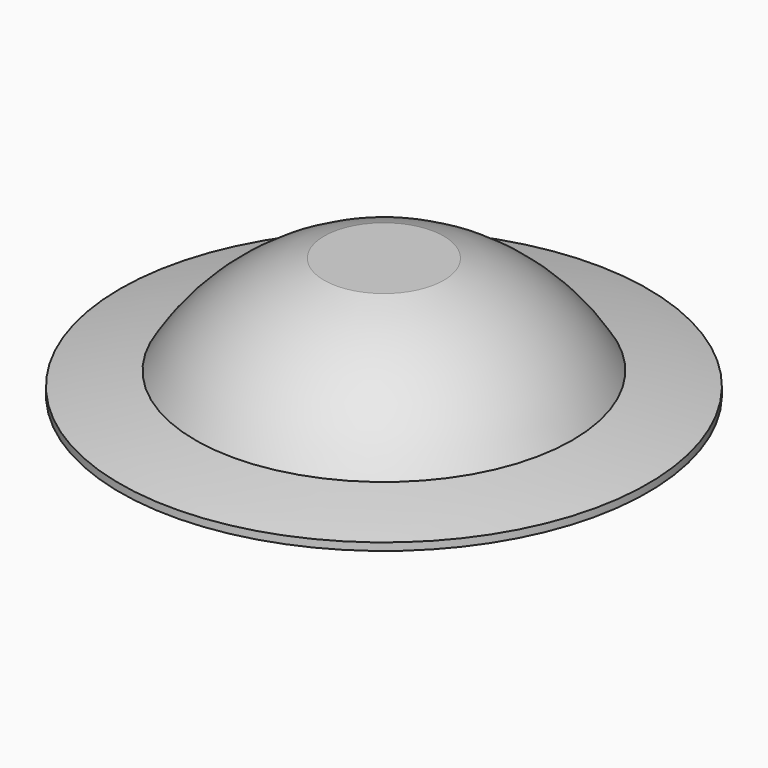
from build123d import *


# Not quite as in the source:
# - ends of sketch curves that miss each other by under 0.0002 mm in the source are joined


with BuildPart() as f1:
    # F0 (on Front) → F1 (revolve)
    with BuildSketch(Plane.XZ):
        with BuildLine():
            ThreePointArc((-6.3500000458, 6.3822891616), (-14.1800115363, 2.4471847578), (-20.0000000206, -4.1042929877))
            ThreePointArc((-20.0000000206, -4.1042929877), (-24.0113747285, -4.7817226312), (-28.0000000016, -5.5822889926))
            Line((-28.0000000016, -5.5822889926), (-28, -6.382289))
            ThreePointArc((-28, -6.382289), (-14.0801278407, -4.1344291551), (0, -3.382289))
            Line((0, -3.382289), (0, 6.382289))
            Line((0, 6.382289), (-6.3500000458, 6.3822891616))
        make_face()
    revolve(axis=Axis((0, 0, 1.5), (0, 0, -1)))


solid = f1.part
